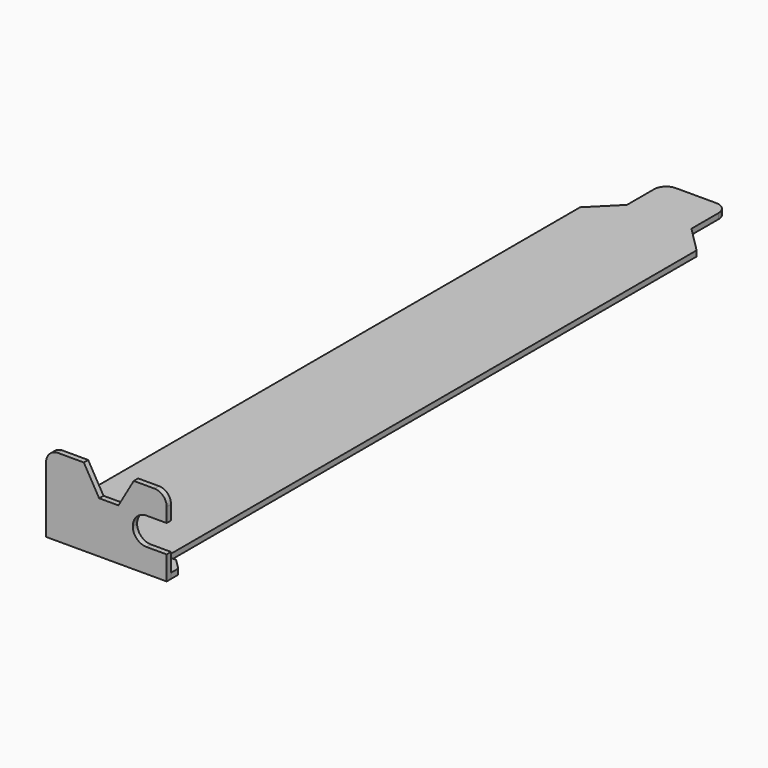
from build123d import *

# Parameters (mm, degrees)
F1_DEPTH = 0.8636
F2_DEPTH = 0.8636
F3_DEPTH = 11.43
F4_W     = 3.048
F4_H     = 4.191
F5_DEPTH = 0.8636


# Not quite as in the source:
# - a feature names something its author has since deleted; it is built from what else it names


with BuildPart() as f1:
    # F0 (on Top) → F1 (new body)
    with BuildSketch(Plane.XY):
        Polygon((10.7315, -58.039), (9.2075, -58.039), (-6.6675, -58.039), (-6.6675, -61.1124), (12.3825, -61.1124), (12.3825, -59.69), align=None)
        with BuildLine():
            ThreePointArc((5.0927, 56.134), (4.5347384182, 57.4810384182), (3.1877, 58.039))
            Line((3.1877, 58.039), (0, 58.039))
            Line((0, 58.039), (-3.1877, 58.039))
            ThreePointArc((-3.1877, 58.039), (-4.5347384182, 57.4810384182), (-5.0927, 56.134))
            Line((-5.0927, 56.134), (-5.0927, 50.7746))
            Line((-5.0927, 50.7746), (-9.2075, 46.6598))
            Line((-9.2075, 46.6598), (-9.2075, -55.499))
            Line((-9.2075, -55.499), (-6.6675, -58.039))
            Line((-6.6675, -58.039), (9.2075, -58.039))
            Line((9.2075, -58.039), (9.2075, 46.6598))
            Line((9.2075, 46.6598), (5.0927, 50.7746))
            Line((5.0927, 50.7746), (5.0927, 56.134))
        make_face()
    extrude(amount=F1_DEPTH)


with BuildPart() as f2:
    # F2 (new): a face of the model
    f2_faces = [f1.part.faces().sort_by_distance(p)[0] for p in [
        (2.8575, -61.1124, 0.4318),
    ]]
    extrude(f2_faces, amount=F2_DEPTH)

    # F3 (add): a face of the model
    f3_faces = [f2.faces().sort_by_distance(p)[0] for p in [
        (2.8575, -61.5442, 0.8636),
    ]]
    extrude(f3_faces, amount=F3_DEPTH)

    # F4 (on face) → F5 (cut)
    with BuildSketch(Plane.XZ.offset(61.976)):
        with BuildLine():
            Line((12.3825, 3.7627826078), (12.3825, 8.1244173922))
            Line((12.3825, 8.1244173922), (9.2075, 8.1244173922))
            ThreePointArc((9.2075, 8.1244173922), (7.6654292335, 7.4856707665), (7.0266826078, 5.9436))
            ThreePointArc((7.0266826078, 5.9436), (7.6654292335, 4.4015292335), (9.2075, 3.7627826078))
            Line((9.2075, 3.7627826078), (12.3825, 3.7627826078))
        make_face()
        Polygon((1.7145, 8.1026), (1.7145, 12.2936), (-0.7051749782, 12.2936), align=None)
        with Locations((3.2385, 10.1981)):
            Rectangle(F4_W, F4_H)
        Polygon((7.1821749782, 12.2936), (4.7625, 12.2936), (4.7625, 8.1026), align=None)
        with BuildLine():
            Line((12.3825, 12.2936), (10.4775, 12.2936))
            ThreePointArc((10.4775, 12.2936), (11.8245384182, 11.7356384182), (12.3825, 10.3886))
            Line((12.3825, 10.3886), (12.3825, 12.2936))
        make_face()
        with BuildLine():
            ThreePointArc((-6.6675, 10.3886), (-6.1095384182, 11.7356384182), (-4.7625, 12.2936))
            Line((-4.7625, 12.2936), (-6.6675, 12.2936))
            Line((-6.6675, 12.2936), (-6.6675, 10.3886))
        make_face()
    extrude(amount=-F5_DEPTH, mode=Mode.SUBTRACT)


solid = Compound([f1.part, f2.part])
